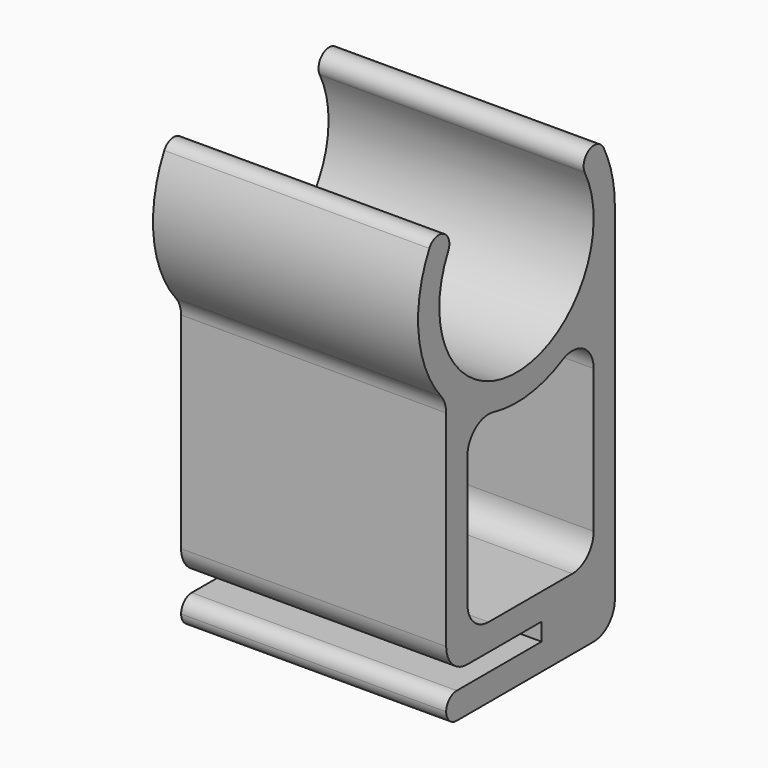
from build123d import *

# Parameters (mm, degrees)
F1_DEPTH = 15
F3_DEPTH = 30
F4_R     = 1.49999
F6_DEPTH = 30.001
F7_R     = 3


# Not quite as in the source:
# - a fillet or chamfer is up to 0.001 mm smaller than in the source, because OpenCascade refuses the exact size


with BuildPart() as f1:
    # F0 (on Right) → F1 (new body, symmetric)
    with BuildSketch(Plane.YZ):
        with BuildLine():
            ThreePointArc((12.3245305001, 6.4665811641), (10.2993352496, 7.0979164137), (9.668, 5.0727211632))
            ThreePointArc((9.668, 5.0727211632), (0, -10.918), (-9.668, 5.0727211632))
            ThreePointArc((-9.668, 5.0727211632), (-10.2993352496, 7.0979164137), (-12.3245305001, 6.4665811641))
            ThreePointArc((-12.3245305001, 6.4665811641), (0, -13.918), (12.3245305001, 6.4665811641))
        make_face()
    extrude(amount=F1_DEPTH, both=True)

    # F2 (on face) → F3 (join, through all)
    with BuildSketch(Plane.YZ.offset(15)):
        with BuildLine():
            ThreePointArc((13.918, 0), (5.2588084202, -12.886258495), (-9.944, -9.7379457793))
            Line((-9.944, -9.7379457793), (-9.944, -37.168))
            Line((-9.944, -37.168), (3.556, -37.168))
            Line((3.556, -37.168), (3.556, -39.168))
            Line((3.556, -39.168), (-9.944, -39.168))
            Line((-9.944, -39.168), (-9.944, -42.168))
            Line((-9.944, -42.168), (13.918, -42.168))
            Line((13.918, -42.168), (13.918, 0))
        make_face()
    extrude(amount=-F3_DEPTH)

    # F4 (radius 1.5 in the source; OpenCascade refuses exactly that, so slightly less here)
    f4_edges = [f1.edges().sort_by_distance(p)[0] for p in [
        (0, -9.944, -39.168),
        (0, -9.944, -42.168),
    ]]
    fillet(f4_edges, radius=F4_R)

    # F5 (on face) → F6 (cut, through all)
    with BuildSketch(Plane.YZ.offset(15)):
        with BuildLine():
            ThreePointArc((10.918, -8.6318016659), (2.6248268424, -13.6682481704), (-6.944, -12.0619893882))
            Line((-6.944, -12.0619893882), (-6.944, -34.168))
            Line((-6.944, -34.168), (10.918, -34.168))
            Line((10.918, -34.168), (10.918, -8.6318016659))
        make_face()
    extrude(amount=-F6_DEPTH, mode=Mode.SUBTRACT)

    # F7
    f7_edges = [f1.edges().sort_by_distance(p)[0] for p in [
        (0, -9.944, -9.737946),
        (0, -9.944, -37.168),
        (0, 13.918, -42.168),
        (0, -6.944, -12.061989),
        (0, 10.918, -8.631802),
        (0, 10.918, -34.168),
        (0, -6.944, -34.168),
    ]]
    fillet(f7_edges, radius=F7_R)


solid = f1.part
